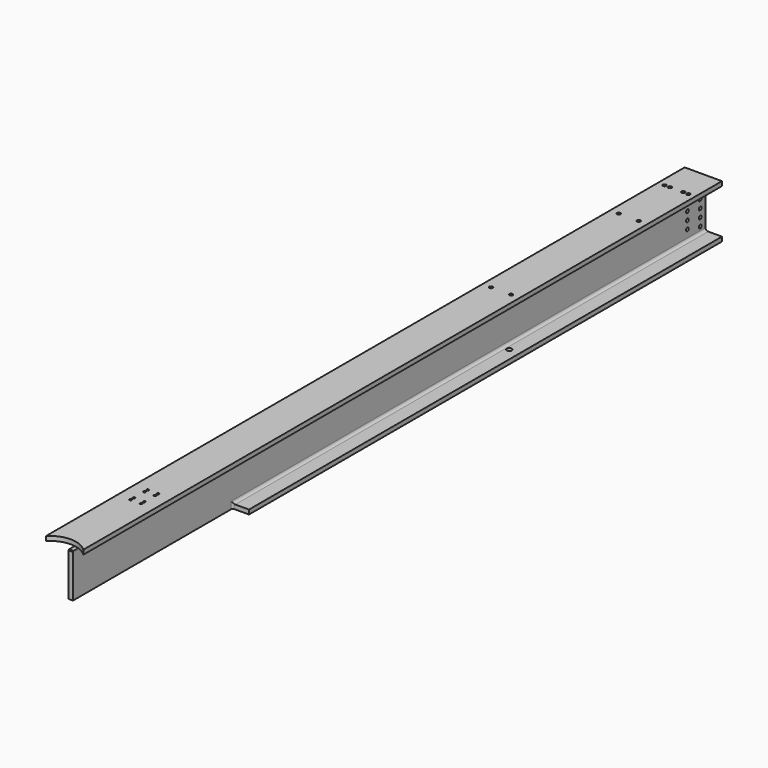
from build123d import *

# Parameters (mm, degrees)
F1_DEPTH  = 1524
F2_R      = 5.08
F4_DEPTH  = 101.6
F6_W      = 48.26
F6_H      = 10.16
F7_DEPTH  = 12.7
F8_SIZE   = 1.27
F10_D     = 4.318
F10_DEPTH = 25.4
F10_TIP   = 1.2972580765
F11_W     = 35.4891605821
F11_H     = 399.7617846188
F12_DEPTH = 25.4
F13_R     = 3.175
F15_D     = 6.5278
F15_DEPTH = 25.4
F15_TIP   = 1.9611489744
F17_D     = 6.5278
F17_DEPTH = 25.4
F17_TIP   = 1.9611489744
F19_D     = 6.5278
F19_DEPTH = 25.4
F19_TIP   = 1.9611489744
F21_D     = 9.8044
F21_DEPTH = 25.4
F21_TIP   = 2.9455389266


with BuildPart() as f1:
    # F0 (on Front) → F1 (new body)
    with BuildSketch(Plane.XZ):
        Polygon((-35.56, -50.8), (35.56, -50.8), (35.56, -42.418), (4.191, -42.418), (4.191, 0), (4.191, 42.418), (35.56, 42.418), (35.56, 50.8), (0, 50.8), (-4.191, 50.8), (-35.56, 50.8), (-35.56, 42.418), (-4.191, 42.418), (-4.191, 0), (-4.191, -42.418), (-35.56, -42.418), align=None)
    extrude(amount=F1_DEPTH)

    # F2
    f2_edges = [f1.edges().sort_by_distance(p)[0] for p in [
        (4.191, -762, 42.418),
        (4.191, -762, -42.418),
        (-4.191, -762, -42.418),
        (-4.191, -762, 42.418),
    ]]
    fillet(f2_edges, radius=F2_R)

    # F3 (on face) → F4 (cut)
    with BuildSketch(Plane.XY.offset(50.8)):
        Polygon((35.56, -1524), (0, -1524), (0, -1560.278456417), align=None)
        with BuildLine():
            Line((0, -1560.278456417), (0, -1524))
            Line((0, -1524), (-35.56, -1524))
            ThreePointArc((-35.56, -1524), (-47.0297011791, -1579.4838516748), (0, -1611.078456417))
            ThreePointArc((0, -1611.078456417), (35.9210244843, -1596.1994809013), (50.8, -1560.278456417))
            ThreePointArc((50.8, -1560.278456417), (46.835285843, -1540.6037010183), (35.56, -1524))
            Line((35.56, -1524), (0, -1560.278456417))
        make_face()
        with BuildLine():
            Line((-35.56, -1524), (0, -1524))
            Line((0, -1524), (35.56, -1524))
            ThreePointArc((35.56, -1524), (0, -1509.478456417), (-35.56, -1524))
        make_face()
    extrude(amount=-F4_DEPTH, mode=Mode.SUBTRACT)

    # F6 (on face) → F7 (cut, symmetric)
    with BuildSketch(Plane.YZ.offset(4.191)):
        with Locations((-1486.2015990684, 37.338)):
            Rectangle(F6_W, F6_H)
    extrude(amount=F7_DEPTH, both=True, mode=Mode.SUBTRACT)

    # F8
    f8_edges = [f1.edges().sort_by_distance(p)[0] for p in [
        (0, -1509.478456, 32.258),
    ]]
    chamfer(f8_edges, length=F8_SIZE)

    # F10
    with Locations(Plane.XY.offset(50.8)):
        with Locations((-10.2286281229, -1353.8202740377), (-10.2286199642, -1346.2002740377), (-10.2286199642, -1320.8002740377), (-10.2286381092, -1313.1802740377), (9.711437429, -1313.1802740377), (9.711419284, -1320.8002740377), (9.711419284, -1346.2002740377), (9.7114274426, -1353.8202740377)):
            Hole(F10_D / 2, depth=F10_DEPTH)
            with Locations((0, 0, -(F10_DEPTH + F10_TIP / 2))):  # 118° drill point
                Cone(0, F10_D / 2, F10_TIP, mode=Mode.SUBTRACT)

    # F11 (on face) → F12 (cut)
    with BuildSketch(Plane(origin=(0, 0, -50.8), x_dir=(1, 0, 0), z_dir=(0, 0, -1))):
        Polygon((4.191, 1528.4134149551), (4.191, 1509.6516303364), (4.191, 1128.6516303364), (39.6801605821, 1128.6516303364), (39.6801605821, 1528.4134149551), align=None)
        with Locations((-21.935580291, 1328.5325226457)):
            Rectangle(F11_W, F11_H)
    extrude(amount=-F12_DEPTH, mode=Mode.SUBTRACT)

    # F13
    f13_edges = [f1.edges().sort_by_distance(p)[0] for p in [
        (4.191, -1128.65163, -44.069),
        (-4.191, -1128.65163, -44.069),
    ]]
    fillet(f13_edges, radius=F13_R)

    # F15
    with Locations(Plane.YZ.offset(4.191)):
        with Locations((-43.18, 22.86), (-43.18, 7.62), (-12.7, 30.48), (-12.7, 15.24), (-12.7, 0), (-12.7, -15.24), (-12.7, -30.48), (-43.18, -7.62), (-43.18, -22.86)):
            Hole(F15_D / 2, depth=F15_DEPTH)
            with Locations((0, 0, -(F15_DEPTH + F15_TIP / 2))):  # 118° drill point
                Cone(0, F15_D / 2, F15_TIP, mode=Mode.SUBTRACT)

    # F17
    with Locations(Plane.XY.offset(50.8)):
        with Locations((-22.858562297, -63.9350753549), (-12.7, -63.76416), (12.7, -63.76416), (22.858562297, -63.9350753549)):
            Hole(F17_D / 2, depth=F17_DEPTH)
            with Locations((0, 0, -(F17_DEPTH + F17_TIP / 2))):  # 118° drill point
                Cone(0, F17_D / 2, F17_TIP, mode=Mode.SUBTRACT)

    # F19
    with Locations(Plane.XY.offset(50.8)):
        with Locations((19.05, -177.8), (-19.05, -177.8), (-19.05, -482.6), (19.05, -482.6)):
            Hole(F19_D / 2, depth=F19_DEPTH)
            with Locations((0, 0, -(F19_DEPTH + F19_TIP / 2))):  # 118° drill point
                Cone(0, F19_D / 2, F19_TIP, mode=Mode.SUBTRACT)

    # F21
    with Locations(Plane(origin=(0, 0, -50.8), x_dir=(1, 0, 0), z_dir=(0, 0, -1))):
        with Locations((15.875, 482.6), (-15.875, 482.6)):
            Hole(F21_D / 2, depth=F21_DEPTH)
            with Locations((0, 0, -(F21_DEPTH + F21_TIP / 2))):  # 118° drill point
                Cone(0, F21_D / 2, F21_TIP, mode=Mode.SUBTRACT)


solid = f1.part
